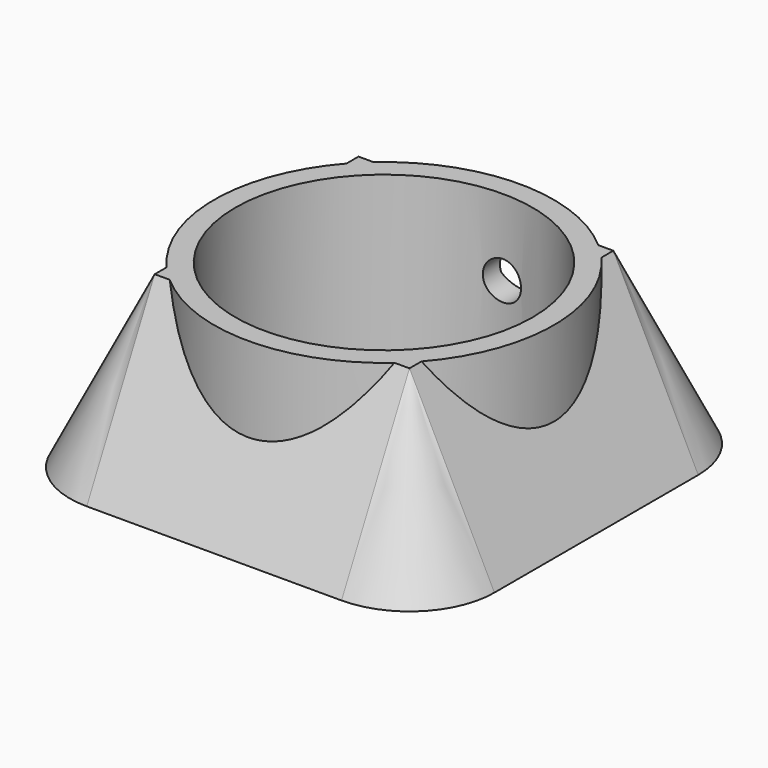
from build123d import *

# Parameters (mm, degrees)
F0_R         = 20
F1_DEPTH     = 20
F2_T1_DEPTH  = 30
F2_T3_DEPTH  = 30
F2_T6_ANGLE  = 90
F2_T8_ANGLE  = 90
F2_T10_ANGLE = 90
F2_T12_ANGLE = 90
F0_R_2       = 17.5
F3_DEPTH     = 20
F4_R         = 2.25
F5_DEPTH     = 25


# Not quite as in the source:
# - a fillet or chamfer that OpenCascade refuses, or shapes differently, is made with other operations: its cross-section is extruded or revolved along the edge and cut away or added


with BuildPart() as f1:
    # F0 (on Top) → F1 (new body)
    with BuildSketch(Plane.XY):
        with BuildLine():
            ThreePointArc((25, 15), (22.0710678119, 22.0710678119), (15, 25))
            Line((15, 25), (-15, 25))
            ThreePointArc((-15, 25), (-22.0710678119, 22.0710678119), (-25, 15))
            Line((-25, 15), (-25, -15))
            ThreePointArc((-25, -15), (-22.0710678119, -22.0710678119), (-15, -25))
            Line((-15, -25), (15, -25))
            ThreePointArc((15, -25), (22.0710678119, -22.0710678119), (25, -15))
            Line((25, -15), (25, 15))
        make_face()
        Circle(F0_R, mode=Mode.SUBTRACT)
    extrude(amount=F1_DEPTH)

    # F2: chamfer of 20 x 10 on 1 edges, made by hand

    # F2_s2 → F2_t1 (cut)
    with BuildSketch(Plane.YZ.offset(-15)):
        Polygon((-25, 0), (-15, 20), (-25, 20), align=None)
        Polygon((25, 0), (15, 20), (25, 20), align=None)
    extrude(amount=F2_T1_DEPTH, mode=Mode.SUBTRACT)

    # F2_s4 → F2_t3 (cut)
    with BuildSketch(Plane.XZ.offset(-15)):
        Polygon((25, 0), (15, 20), (25, 20), align=None)
        Polygon((-25, 0), (-15, 20), (-25, 20), align=None)
    extrude(amount=F2_T3_DEPTH, mode=Mode.SUBTRACT)

    # F2_s5 → F2_t6 (revolve, cut)
    with BuildSketch(Plane.XZ.offset(15)):
        Polygon((-25, 0), (-15, 20), (-25, 20), align=None)
    revolve(axis=Axis((-15, -15, 20), (0, 0, 1)), revolution_arc=F2_T6_ANGLE, mode=Mode.SUBTRACT)

    # F2_s7 → F2_t8 (revolve, cut)
    with BuildSketch(Plane.YZ.offset(15)):
        Polygon((-25, 0), (-15, 20), (-25, 20), align=None)
    revolve(axis=Axis((15, -15, 20), (0, 0, 1)), revolution_arc=F2_T8_ANGLE, mode=Mode.SUBTRACT)

    # F2_s9 → F2_t10 (revolve, cut)
    with BuildSketch(Plane.XZ.offset(-15)):
        Polygon((25, 0), (15, 20), (25, 20), align=None)
    revolve(axis=Axis((15, 15, 20), (0, 0, 1)), revolution_arc=F2_T10_ANGLE, mode=Mode.SUBTRACT)

    # F2_s11 → F2_t12 (revolve, cut)
    with BuildSketch(Plane.YZ.offset(-15)):
        Polygon((25, 0), (15, 20), (25, 20), align=None)
    revolve(axis=Axis((-15, 15, 20), (0, 0, 1)), revolution_arc=F2_T12_ANGLE, mode=Mode.SUBTRACT)

    # F0 (on Top) → F3 (join)
    with BuildSketch(Plane.XY):
        Circle(F0_R)
        Circle(F0_R_2, mode=Mode.SUBTRACT)
    extrude(amount=F3_DEPTH)

    # F4 (on Front) → F5 (cut)
    with BuildSketch(Plane.XZ):
        with Locations((0, 11)):
            Circle(F4_R)
    extrude(amount=-F5_DEPTH, mode=Mode.SUBTRACT)


solid = f1.part
